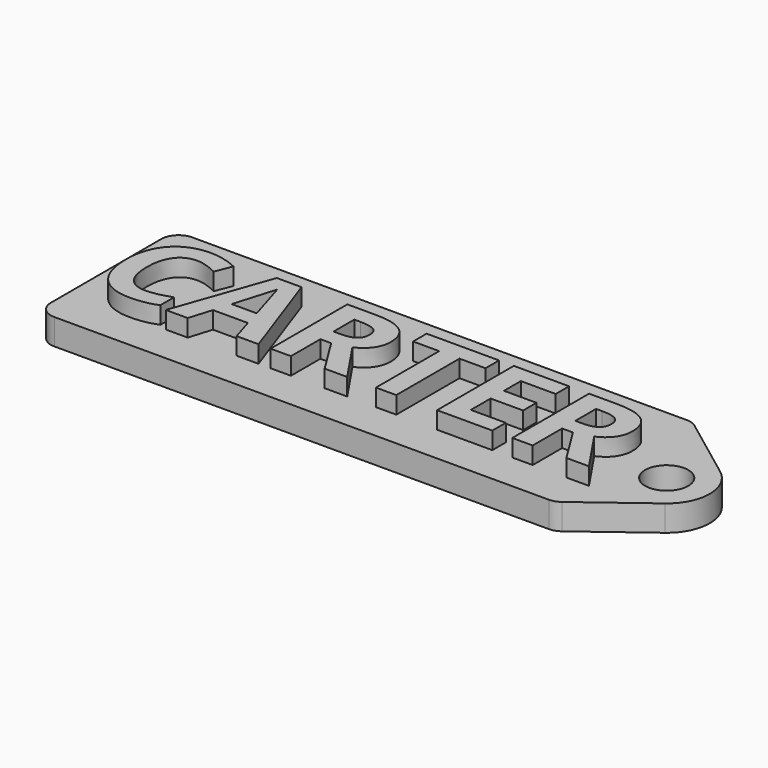
from build123d import *

# Parameters (mm, degrees)
F0_R         = 2.5
F1_DEPTH     = 3
F2_TEXT_SIZE = 15.5787253033
F3_DEPTH     = 2


# Not quite as in the source:
# - Text() gives the source's letters only with a copy of the font that has no kerning and outlines rounded to 1/6400 em; it was checked with that copy


with BuildPart() as f1:
    # F0 (on Top) → F1 (new body)
    with BuildSketch(Plane.XY):
        with BuildLine():
            Line((-28, -10), (29.3333333333, -10))
            ThreePointArc((29.3333333333, -10), (29.9657888654, -9.8973665961), (30.5333333333, -9.6))
            Line((30.5333333333, -9.6), (38, -4))
            ThreePointArc((38, -4), (39.472135955, -2.2360679775), (40, 0))
            ThreePointArc((40, 0), (39.472135955, 2.2360679775), (38, 4))
            Line((38, 4), (30.5333333333, 9.6))
            ThreePointArc((30.5333333333, 9.6), (29.9657888654, 9.8973665961), (29.3333333333, 10))
            Line((29.3333333333, 10), (-28, 10))
            ThreePointArc((-28, 10), (-29.4142135624, 9.4142135624), (-30, 8))
            Line((-30, 8), (-30, -8))
            ThreePointArc((-30, -8), (-29.4142135624, -9.4142135624), (-28, -10))
        make_face()
        with Locations((35, 0)):
            Circle(F0_R, mode=Mode.SUBTRACT)
    extrude(amount=F1_DEPTH)

    # F2 (on face) → F3 (join)
    with BuildSketch(Plane.XY.offset(3)):
        with Locations((-28.5173784941, -5.6083411092)):
            Text('CARTER', F2_TEXT_SIZE, font='Open Sans', font_style=FontStyle.BOLD, text_align=(TextAlign.LEFT, TextAlign.BOTTOM))
    extrude(amount=F3_DEPTH)


solid = f1.part
